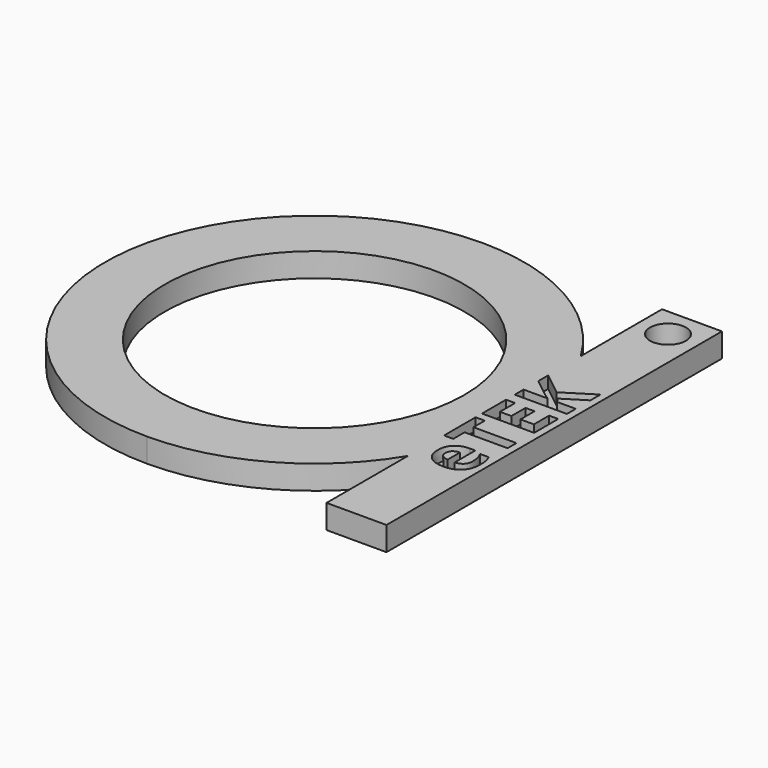
from build123d import *

# Parameters (mm, degrees)
F0_R         = 12.5
F1_DEPTH     = 2
F2_R         = 1.5
F3_DEPTH     = 2
F4_TEXT_SIZE = 6.1006609049
F5_DEPTH     = 1


# Not quite as in the source:
# - Text() gives the source's letters only with a copy of the font that has no kerning and outlines rounded to 1/6400 em; it was checked with that copy


with BuildPart() as f1:
    # F0 (on Top) → F1 (new body)
    with BuildSketch(Plane.XY):
        with BuildLine():
            ThreePointArc((14.9999978021, 9.0138818462), (8.6170490219, 15.2314302071), (0, 17.5))
            ThreePointArc((0, 17.5), (-17.5, 0), (0, -17.5))
            ThreePointArc((0, -17.5), (8.6170490219, -15.2314302071), (14.9999978021, -9.0138818462))
            Line((14.9999978021, -9.0138818462), (14.9999978021, 9.0138818462))
        make_face()
        Circle(F0_R, mode=Mode.SUBTRACT)
        with BuildLine():
            ThreePointArc((17.5, 0), (16.8634213838, 4.6770737894), (14.9999978021, 9.0138818462))
            Line((14.9999978021, 9.0138818462), (14.9999978021, -9.0138818462))
            ThreePointArc((14.9999978021, -9.0138818462), (16.8634213838, -4.6770737894), (17.5, 0))
        make_face()
        with BuildLine():
            Line((14.9999978021, 17.4999999255), (14.9999978021, 9.0138818462))
            ThreePointArc((14.9999978021, 9.0138818462), (16.8634213838, 4.6770737894), (17.5, 0))
            ThreePointArc((17.5, 0), (16.8634213838, -4.6770737894), (14.9999978021, -9.0138818462))
            Line((14.9999978021, -9.0138818462), (14.9999978021, -17.5000000745))
            Line((14.9999978021, -17.5), (19.9999978021, -17.5))
            Line((19.9999978021, -17.5000000745), (19.9999978021, 17.4999999255))
            Line((19.9999978021, 17.5), (14.9999978021, 17.5))
        make_face()
    extrude(amount=F1_DEPTH)

    # F2 (on face) → F3 (cut)
    with BuildSketch(Plane.XY.offset(2)):
        with Locations((17.4999963492, 15.0000024587)):
            Circle(F2_R)
    extrude(amount=-F3_DEPTH, mode=Mode.SUBTRACT)

    # F4 (on face) → F5 (cut)
    with BuildSketch(Plane.XY.offset(2)):
        with Locations(Location((19.3924736536, -9.0138819069), (0, 0, 90))):
            Text('eTEK', F4_TEXT_SIZE, font='Open Sans', font_style=FontStyle.BOLD, text_align=(TextAlign.LEFT, TextAlign.BOTTOM))
    extrude(amount=-F5_DEPTH, mode=Mode.SUBTRACT)


solid = f1.part
